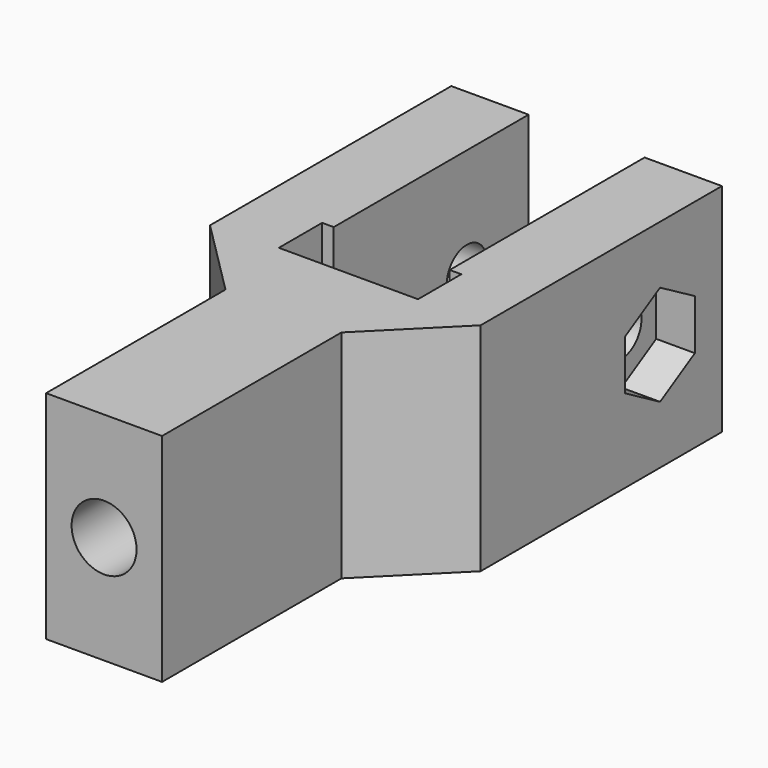
from build123d import *

# Parameters (mm, degrees)
F1_DEPTH  = 14
F2_R      = 2.1
F3_DEPTH  = 25
F5_W      = 9
F5_H      = 3.5
F6_DEPTH  = 10
F4_R      = 2.1
F7_DEPTH  = 1.75
F8_R      = 1.625
F9_DEPTH  = 2.5
F10_DEPTH = 25
F11_R     = 2.85
F11_R_2   = 1.625
F12_DEPTH = 2


with BuildPart() as f1:
    # F0 (on Top) → F1 (new body)
    with BuildSketch(Plane.XY):
        Polygon((5, 0), (0, 0), (0, -19.5), (5, -24.5), (5, -39), (12.5, -39), (12.5, -24.5), (17.5, -19.5), (17.5, 0), (12.5, 0), (12.5, -17.5), (5, -17.5), align=None)
    extrude(amount=F1_DEPTH)

    # F2 (on face) → F3 (cut)
    with BuildSketch(Plane.XZ.offset(39)):
        with Locations((8.75, 7)):
            Circle(F2_R)
    extrude(amount=-F3_DEPTH, mode=Mode.SUBTRACT)

    # F5 (on face) → F6 (cut)
    with BuildSketch(Plane.XY.offset(14)):
        with Locations((8.75, -17.5)):
            Rectangle(F5_W, F5_H)
    extrude(amount=-F6_DEPTH, mode=Mode.SUBTRACT)

    # F4 (on face) → F7 (cut)
    with BuildSketch(Plane(origin=(0, -17.5, 0), x_dir=(-1, 0, 0), z_dir=(0, 1, 0))):
        Polygon((-5, 4.2150635095), (-5, 9.7849364905), (-8.75, 11.95), (-12.5, 9.7849364905), (-12.5, 4.2150635095), (-8.75, 2.05), align=None)
        with Locations((-8.75, 7)):
            Circle(F4_R, mode=Mode.SUBTRACT)
    extrude(amount=-F7_DEPTH, mode=Mode.SUBTRACT)

    # F8 (on face) → F9 (cut)
    with BuildSketch(Plane.YZ.offset(17.5)):
        Polygon((-2.1854174377, 5.375), (-2.1854174377, 8.625), (-5, 10.25), (-7.8145825623, 8.625), (-7.8145825623, 5.375), (-5, 3.75), align=None)
        with Locations((-5, 7)):
            Circle(F8_R, mode=Mode.SUBTRACT)
    extrude(amount=-F9_DEPTH, mode=Mode.SUBTRACT)

    # F10 (cut): a face of the model
    f10_faces = [f1.faces().sort_by_distance(p)[0] for p in [
        (17.5, -5, 7),
    ]]
    extrude(f10_faces, amount=-F10_DEPTH, mode=Mode.SUBTRACT)

    # F11 (on face) → F12 (cut)
    with BuildSketch(Plane(origin=(0, 0, 0), x_dir=(0, -1, 0), z_dir=(-1, 0, 0))):
        with Locations((5, 7)):
            Circle(F11_R)
        with Locations((5, 7)):
            Circle(F11_R_2, mode=Mode.SUBTRACT)
    extrude(amount=-F12_DEPTH, mode=Mode.SUBTRACT)


solid = f1.part
